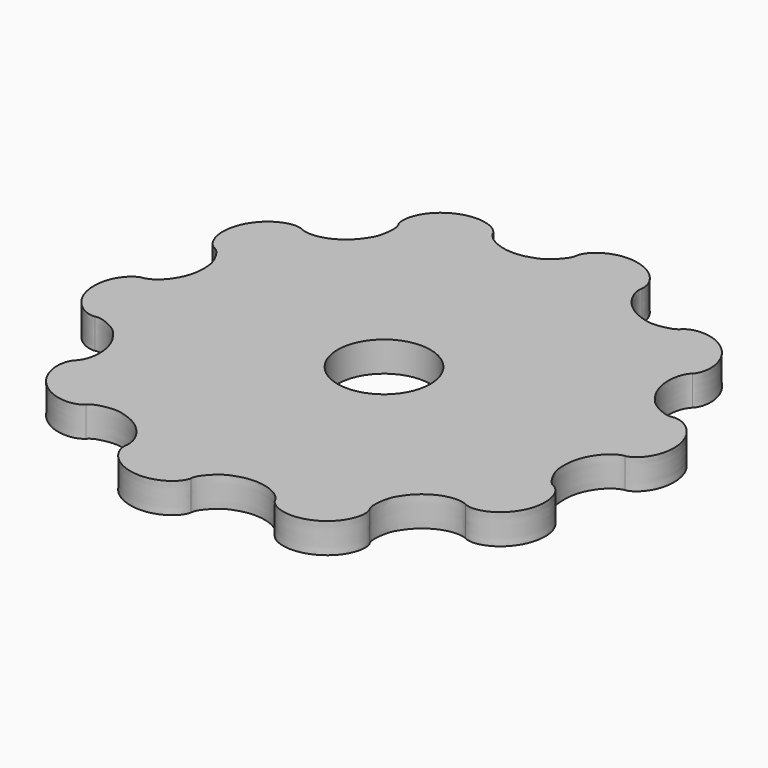
from build123d import *

# Parameters (mm, degrees)
F1_R            = 20
F2_DEPTH        = 2.5
F4_DEPTH        = 2.5
F4_COPIES_COUNT = 10
F6_DEPTH        = 2.5010001
F6_COPIES_COUNT = 10
F7_R            = 3.85
F8_DEPTH        = 2.5010001


# Not quite as in the source:
# - a pattern or mirror of a feature is missing from the dataset's text; its kind, count and spacing are read off the source's solid


with BuildPart() as f2:
    # F1 (on Top) → F2 (new body)
    with BuildSketch(Plane.XY):
        Circle(F1_R)
    extrude(amount=F2_DEPTH)

    # F3 (on face) → F4 (join, through all)
    with BuildSketch(Plane.XY.offset(2.5)):
        with BuildLine():
            add(Edge.make_bspline(
                [(19.0211303259, 6.1803398875), (19.0686831517, 6.1957907372), (19.1689214219, 6.2040348517), (19.6159715324, 6.1646497501), (20.2175106235, 5.8961877736), (20.8933965846, 5.338911141), (21.4572246926, 4.4925295632), (21.7814913502, 3.4498489196), (21.7953013047, 2.3579976194), (21.5206151899, 1.3788083296), (21.0500176404, 0.6399466184), (20.5608785082, 0.1987381116), (20.1478832259, 0.0231358894), (20.0499999874, 0), (20, 3.54743e-05)],
                knots=[0, 0, 0, 0, 0.0392243166, 0.1063522461, 0.1910143777, 0.2876626697, 0.3919584486, 0.5000004826, 0.6080424797, 0.7123382586, 0.8089865505, 0.8936486822, 0.9607766117, 1, 1, 1, 1], degree=3))
            ThreePointArc((19.0211303259, 6.1803398875), (19.1003988891, 5.9308314995), (19.1763946974, 5.6803068941))
            ThreePointArc((19.1763946974, 5.6803068941), (19.2491047291, 5.4288089973), (19.3185165258, 5.176380902))
            ThreePointArc((19.3185165258, 5.176380902), (19.8288949123, 2.6105414298), (20, 3.54743e-05))
        make_face()
    f4 = extrude(amount=-F4_DEPTH)

    # F4_copies: F4 ×10 about axis
    f4_copies_axis = Axis((0, 0, 0), (0, 0, 1))
    for i in range(1, F4_COPIES_COUNT):
        add(f4.rotate(f4_copies_axis, i * 360 / F4_COPIES_COUNT))

    # F5 (on face) → F6 (cut, through all)
    with BuildSketch(Plane.XY.offset(2.5)):
        with BuildLine():
            ThreePointArc((16.4825237724, 11.3281247385), (16.3328311032, 11.5429038007), (16.1803398875, 11.7557050458))
            add(Edge.make_bspline(
                [(19.0211303259, 6.1803398875), (18.9735775001, 6.1648890378), (18.8833193536, 6.1609410802), (18.4645271896, 6.1217292519), (17.1742773102, 6.6910456531), (16.5803863442, 7.3249170155), (15.9950963404, 8.1569427328), (15.6649480183, 9.0772565217), (15.5532672544, 9.9883091577), (15.6502850404, 10.7731352472), (15.8470729584, 11.3306356791), (16.0851016337, 11.6653608233), (16.1398890378, 11.7263157832), (16.1803398875, 11.7557050458)],
                knots=[0, 0, 0, 0, 0.0414235536, 0.1123272793, 0.2475899302, 0.3577541603, 0.4718755225, 0.5859967913, 0.6961610214, 0.7982473204, 0.8876727207, 0.9585764464, 1, 1, 1, 1], degree=3))
            ThreePointArc((19.0211303259, 6.1803398875), (17.9374548307, 8.8457738044), (16.4825237724, 11.3281247385))
        make_face()
    f6 = extrude(amount=-F6_DEPTH, mode=Mode.SUBTRACT)

    # F6_copies: F6 ×10 about axis
    f6_copies_axis = Axis((0, 0, 0), (0, 0, 1))
    for i in range(1, F6_COPIES_COUNT):
        add(f6.rotate(f6_copies_axis, i * 360 / F6_COPIES_COUNT), mode=Mode.SUBTRACT)

    # F7 (on face) → F8 (cut, through all)
    with BuildSketch(Plane.XY.offset(2.5)):
        Circle(F7_R)
    extrude(amount=-F8_DEPTH, mode=Mode.SUBTRACT)


solid = f2.part
